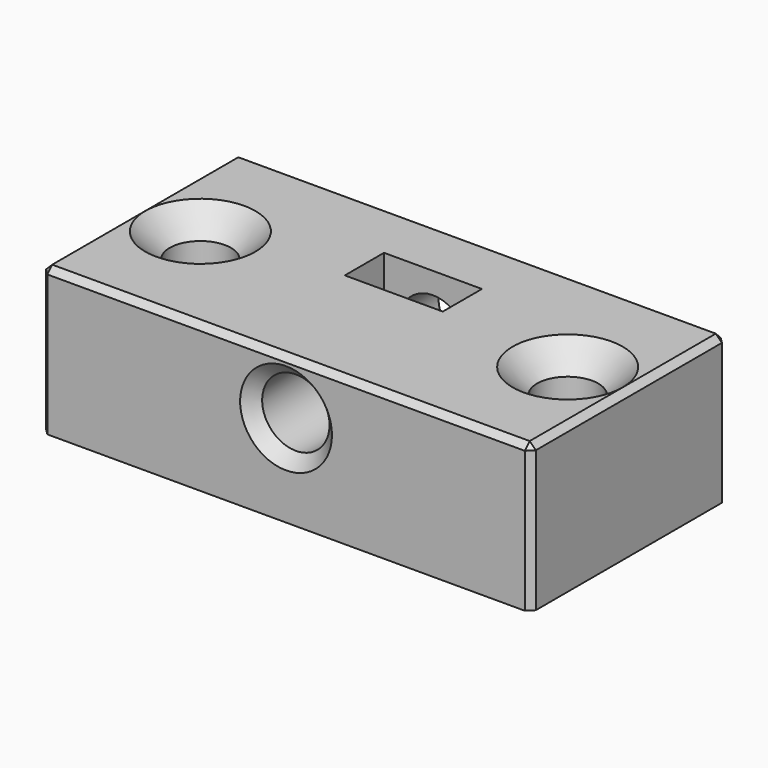
from build123d import *

# Parameters (mm, degrees)
F0_W     = 40
F0_H     = 20
F0_R     = 2.5
F0_W_2   = 8
F0_H_2   = 4
F1_DEPTH = 12
F2_DEPTH = 3
F3_R     = 2.75
F4_DEPTH = 25
F5_SIZE  = 2
F6_SIZE  = 1
F7_SIZE  = 0.49999


# Not quite as in the source:
# - a fillet or chamfer is up to 0.001 mm smaller than in the source, because OpenCascade refuses the exact size


with BuildPart() as f1:
    # F0 (on Top) → F1 (new body)
    with BuildSketch(Plane.XY):
        Rectangle(F0_W, F0_H)
        with Locations((-15, 0)):
            Circle(F0_R, mode=Mode.SUBTRACT)
        with Locations((0, 3)):
            Rectangle(F0_W_2, F0_H_2, mode=Mode.SUBTRACT)
        with Locations((15, 0)):
            Circle(F0_R, mode=Mode.SUBTRACT)
    extrude(amount=F1_DEPTH)

    # F0 (on Top) → F2 (join)
    with BuildSketch(Plane.XY):
        with Locations((0, 3)):
            Rectangle(F0_W_2, F0_H_2)
    extrude(amount=F2_DEPTH)

    # F3 (on face) → F4 (cut)
    with BuildSketch(Plane.XZ.offset(10)):
        with Locations((0, 7.5)):
            Circle(F3_R)
    extrude(amount=-F4_DEPTH, mode=Mode.SUBTRACT)

    # F5
    f5_edges = [f1.edges().sort_by_distance(p)[0] for p in [
        (-17.5, 0, 12),
        (12.5, 0, 12),
    ]]
    chamfer(f5_edges, length=F5_SIZE)

    # F6
    f6_edges = [f1.edges().sort_by_distance(p)[0] for p in [
        (-2.75, 10, 7.5),
        (-17.5, 0, 0),
        (12.5, 0, 0),
        (-2.75, -10, 7.5),
    ]]
    chamfer(f6_edges, length=F6_SIZE)

    # F7 (size 0.5 in the source; OpenCascade refuses exactly that, so slightly less here)
    f7_edges = [f1.edges().sort_by_distance(p)[0] for p in [
        (0, 10, 12),
        (20, 0, 12),
        (0, -10, 12),
        (-20, 0, 12),
        (-20, 10, 6),
        (20, 10, 6),
        (20, -10, 6),
        (-20, -10, 6),
    ]]
    chamfer(f7_edges, length=F7_SIZE)


solid = f1.part
